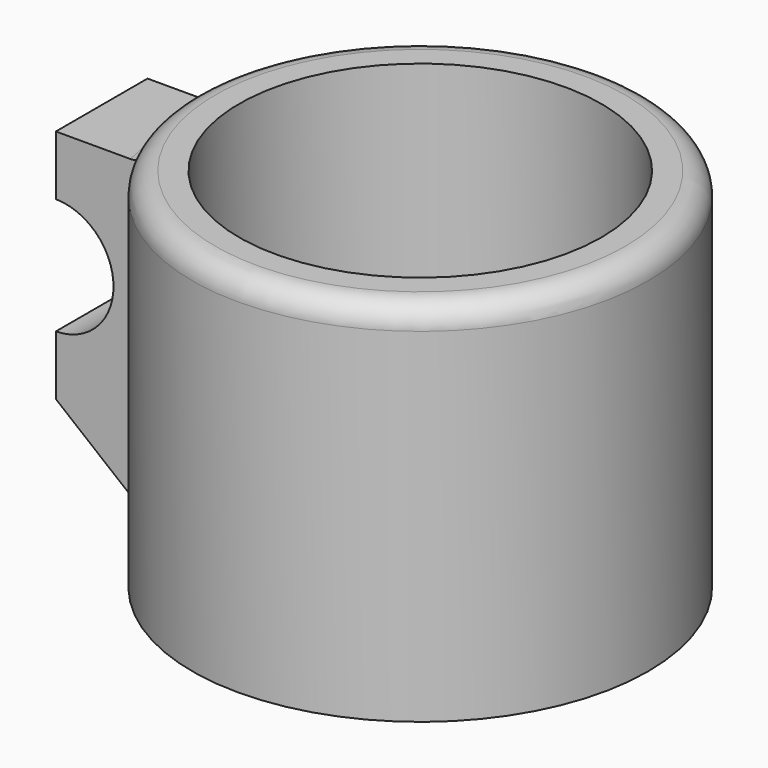
from build123d import *

# Parameters (mm, degrees)
F1_DEPTH       = 12.5
F2_R           = 49.7287092038
F3_DEPTH       = 70
F5_DEPTH       = 10
F8_D           = 26
F8_CBORE_D     = 79
F8_CBORE_DEPTH = 60
F9_R           = 5
F10_R          = 4.99999


# Not quite as in the source:
# - a fillet or chamfer is up to 0.001 mm smaller than in the source, because OpenCascade refuses the exact size
# - a feature names something its author has since deleted; it is built from what else it names


with BuildPart() as f1:
    # F0 (on Front) → F1 (new body, symmetric)
    with BuildSketch(Plane.XZ):
        with BuildLine():
            Line((0, -70), (0, 0))
            Line((0, 0), (-23, 0))
            Line((-23, 0), (-23, -13))
            ThreePointArc((-23, -13), (-10.4224046937, -25.699410108), (-23, -38.398820216))
            Line((-23, -38.398820216), (-23, -51.398820216))
            Line((-23, -51.398820216), (0, -70))
        make_face()
    extrude(amount=F1_DEPTH, both=True)

    # F2 (on Top) → F3 (join)
    with BuildSketch(Plane.XY):
        with Locations((46.5068519115, 0)):
            Circle(F2_R)
    extrude(amount=-F3_DEPTH)

    # F2 (on Top) → F5 (join)
    with BuildSketch(Plane.XY):
        with Locations((46.5068519115, 0)):
            Circle(F2_R)
    extrude(amount=F5_DEPTH)

    # F8 (through all)
    with Locations(Plane.XY.offset(10)):
        with Locations((46.5068519115, 0)):
            CounterBoreHole(F8_D / 2, F8_CBORE_D / 2, F8_CBORE_DEPTH)

    # F9
    f9_edges = [f1.edges().sort_by_distance(p)[0] for p in [
        (-3.221857, 0, 10),
    ]]
    fillet(f9_edges, radius=F9_R)

    # F10 (radius 5 in the source; OpenCascade refuses exactly that, so slightly less here)
    f10_edges = [f1.edges().sort_by_distance(p)[0] for p in [
        (-1.625201, 12.5, -34.342812),
        (-1.625201, -12.5, -34.342812),
        (-3.221857, 0, 0),
    ]]
    fillet(f10_edges, radius=F10_R)


solid = f1.part
